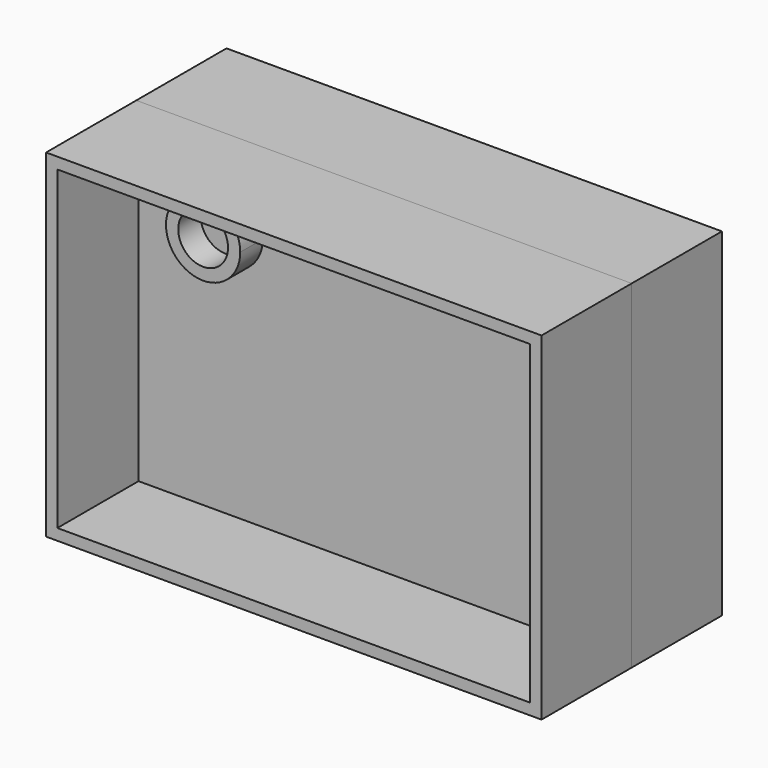
from build123d import *

# Parameters (mm, degrees)
F0_W     = 87.8789871931
F0_H     = 59.9904470146
F1_DEPTH = 20
F2_T     = -2
F3_R     = 4.4185706022
F4_DEPTH = 25
F5_DEPTH = 20
F6_W     = 87.8789871931
F6_H     = 59.9904470146
F7_DEPTH = 20
F8_T     = -2


# Not quite as in the source:
# - ends of sketch curves that miss each other by under 0.0002 mm in the source are joined


with BuildPart() as f1:
    # F0 (on Front) → F1 (new body)
    with BuildSketch(Plane.XZ):
        Rectangle(F0_W, F0_H)
    extrude(amount=-F1_DEPTH)

    # F2
    f2_openings = [f1.faces().sort_by_distance(p)[0] for p in [
        (0, 0, 0),
    ]]
    offset(amount=F2_T, openings=f2_openings)

    # F3 (on face) → F4 (join)
    with BuildSketch(Plane.XZ.offset(-18)):
        with BuildLine():
            ThreePointArc((-32.6843762426, 14.7468157928), (-25.3642450586, 10.4684114553), (-19.9026966179, 16.9538222253))
            ThreePointArc((-19.9026966179, 16.9538222253), (-25.3642446263, 23.4392329207), (-32.6843759484, 19.1608294845))
            ThreePointArc((-32.6843759484, 19.1608294845), (-33.0654589748, 16.953822664), (-32.6843762426, 14.7468157928))
        make_face()
        with Locations((-26.4840777963, 16.9538222253)):
            Circle(F3_R, mode=Mode.SUBTRACT)
    extrude(amount=F4_DEPTH)

    # F3 (on face) → F5 (join)
    with BuildSketch(Plane.XZ.offset(-18)):
        with BuildLine():
            ThreePointArc((-32.6843762426, 14.7468157928), (-33.0654589748, 16.953822664), (-32.6843759484, 19.1608294845))
            Line((-32.6843759484, 19.1608294845), (-41.9394935966, 19.1608294845))
            Line((-41.9394935966, 19.1608294845), (-41.9394935966, 14.7468158975))
            Line((-41.9394935966, 14.7468158975), (-32.6843762426, 14.7468157928))
        make_face()
    extrude(amount=F5_DEPTH)


with BuildPart() as f7:
    # F6 (on Front) → F7 (new body)
    with BuildSketch(Plane.XZ):
        Rectangle(F6_W, F6_H)
    extrude(amount=F7_DEPTH)

    # F8
    f8_openings = [f7.faces().sort_by_distance(p)[0] for p in [
        (0, -20, 0),
    ]]
    offset(amount=F8_T, openings=f8_openings)


solid = Compound([f1.part, f7.part])
